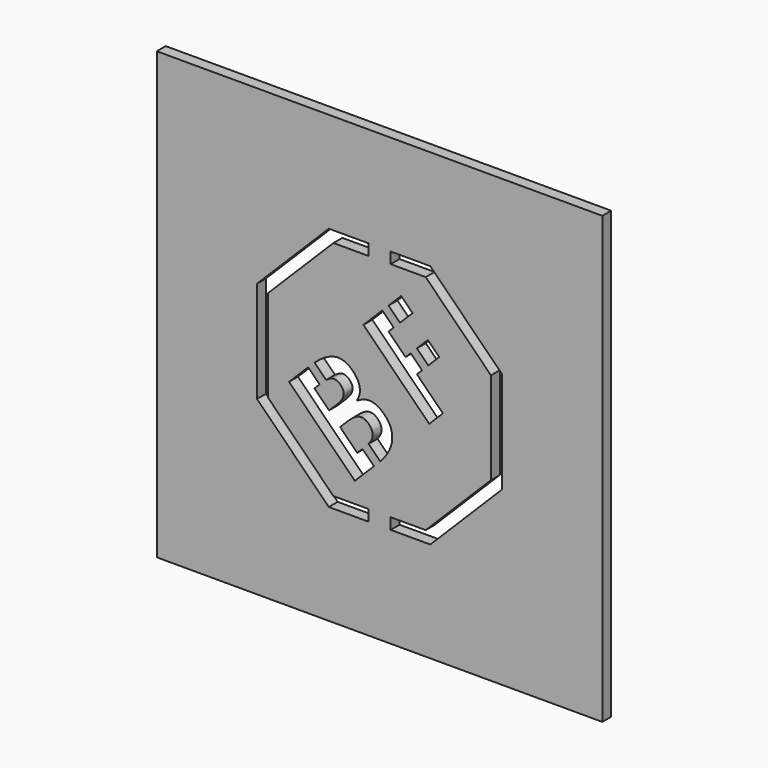
from build123d import *

# Parameters (mm, degrees)
F0_W           = 127
F0_H           = 127
F1_DEPTH       = 3.175
F3_DEPTH       = 3.175
F4_TEXT_SIZE   = 37.1311100959
F4_TEXT_SIZE_2 = 37.1475
F5_DEPTH       = 3.175
F7_DEPTH       = 3.175


# Not quite as in the source:
# - Text() gives the source's letters only with a copy of the font that has no kerning and outlines rounded to 1/6400 em; it was checked with that copy


with BuildPart() as f1:
    # F0 (on Front) → F1 (new body)
    with BuildSketch(Plane.XZ):
        Rectangle(F0_W, F0_H)
    extrude(amount=-F1_DEPTH)

    # F2 (on face) → F3 (cut, through all)
    with BuildSketch(Plane.XZ):
        Polygon((31.75, -13.1512806053), (13.1512806053, -31.75), (3.175, -31.75), (3.175, -34.925), (14.4664086659, -34.925), (34.925, -14.4664086659), (34.925, 14.4664086659), (14.4664086659, 34.925), (3.175, 34.925), (3.175, 31.75), (13.1512806053, 31.75), (31.75, 13.1512806053), align=None)
        Polygon((-3.175, -31.75), (-13.1512806053, -31.75), (-31.75, -13.1512806053), (-31.75, 13.1512806053), (-13.1512806053, 31.75), (-3.175, 31.75), (-3.175, 34.925), (-14.4664086659, 34.925), (-34.925, 14.4664086659), (-34.925, -14.4664086659), (-14.4664086659, -34.925), (-3.175, -34.925), align=None)
    extrude(amount=-F3_DEPTH, mode=Mode.SUBTRACT)

    # F4 (on face) → F5 (cut, through all)
    with BuildSketch(Plane.XZ):
        with Locations(Location((-9.4065003472, -28.3105753613), (0, 0, 45))):
            Text('B', F4_TEXT_SIZE, font='Open Sans', font_style=FontStyle.BOLD, text_align=(TextAlign.LEFT, TextAlign.BOTTOM))
        with Locations(Location((11.791076287, -7.121343104), (0, 0, 45))):
            Text('F', F4_TEXT_SIZE_2, font='Open Sans', font_style=FontStyle.BOLD, text_align=(TextAlign.LEFT, TextAlign.BOTTOM))
    extrude(amount=-F5_DEPTH, mode=Mode.SUBTRACT)

    # F6 (on face) → F7 (join, through all)
    with BuildSketch(Plane.XZ):
        Polygon((-21.4377847748, -0.6592349397), (-20.3405519378, -1.7564677768), (-13.7265865939, -8.3704331207), (-11.9305353697, -6.5743818964), (-18.5049172662, 0), (-19.6283678524, 1.1501819827), align=None)
        Polygon((-7.0157445121, -11.489172754), (-8.8117957363, -13.2852239782), (-1.5964723502, -20.5005473643), (-0.7209155025, -21.376104212), (1.5552275566, -19.1965709689), (0.1975683052, -18.7024855713), align=None)
        Polygon((2.5692477683, 21.1615350602), (0.7731965441, 19.365483836), (13.4714587612, 6.667221619), (15.2675099854, 8.4632728432), align=None)
    extrude(amount=-F7_DEPTH)


solid = f1.part
